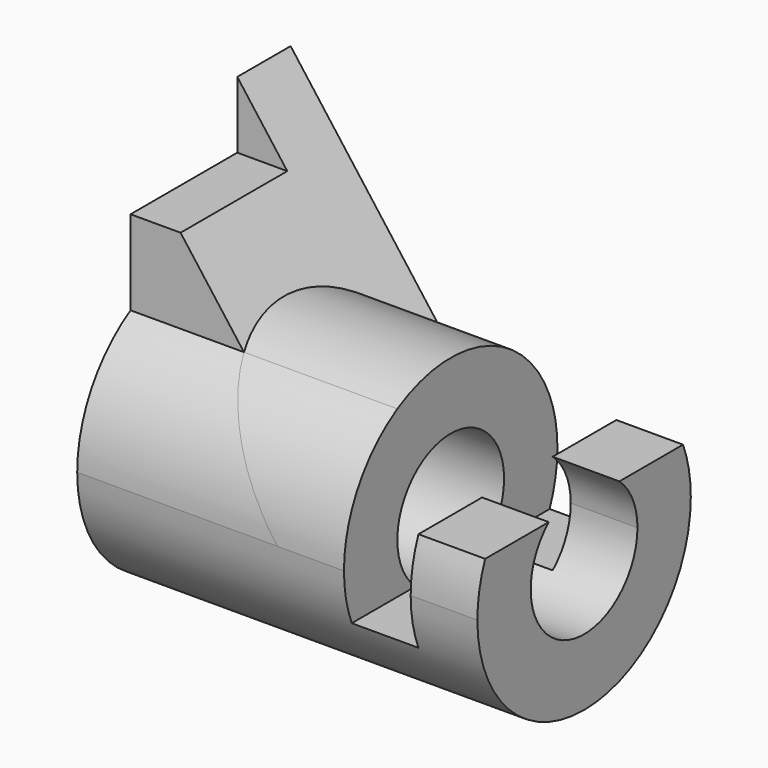
from build123d import *
from build123d import SkipClean  # not in build123d's __all__

# Parameters (mm, degrees)
F0_R      = 25.4
F1_DEPTH  = 76.2
F3_DEPTH  = 25.4
F4_W      = 12.7
F4_H      = 50.8
F5_DEPTH  = 19.05
F7_DEPTH  = 25.4
F8_R      = 12.7
F9_DEPTH  = 76.201
F11_DEPTH = 76.201
F12_W     = 25.4
F12_H     = 12.7
F13_DEPTH = 76.201


with BuildPart() as f1:
    # F0 (on Right) → F1 (new body)
    with BuildSketch(Plane.YZ):
        Circle(F0_R)
    extrude(amount=-F1_DEPTH)

    # F2 (on face) → F3 (cut)
    with BuildSketch(Plane.YZ):
        with BuildLine():
            ThreePointArc((23.5464301965, 9.525), (0, 25.4), (-23.5464301965, 9.525))
            Line((-23.5464301965, 9.525), (23.5464301965, 9.525))
        make_face()
    extrude(amount=-F3_DEPTH, mode=Mode.SUBTRACT)

    # F4 (on face) → F5 (cut)
    with BuildSketch(Plane.XY.offset(9.525)):
        with Locations((-19.05, 0)):
            Rectangle(F4_W, F4_H)
    extrude(amount=-F5_DEPTH, mode=Mode.SUBTRACT)

    # F6 (on Front) → F7 (join, symmetric)
    with BuildSketch(Plane.XZ):
        Polygon((-76.2, 0), (-38.1, 0), (-54.76875, 22.225), (-76.2, 22.225), align=None)
        Polygon((-76.2, 22.225), (-54.76875, 22.225), (-76.2, 50.8), align=None)
    extrude(amount=F7_DEPTH, both=True)

    # F8 (on Right) → F9 (cut, through all)
    with BuildSketch(Plane.YZ):
        Circle(F8_R)
    extrude(amount=-F9_DEPTH, mode=Mode.SUBTRACT)

    # F10 (on face) → F11 (cut, through all)
    with BuildSketch(Plane.YZ):
        with BuildLine():
            ThreePointArc((-25.4, 0), (-21.9970452561, 12.7), (-12.7, 21.9970452561))
            Line((-12.7, 21.9970452561), (-12.7, 50.8))
            Line((-12.7, 50.8), (-25.4, 50.8))
            Line((-25.4, 50.8), (-25.4, 0))
        make_face()
    with SkipClean():  # cleaning this boolean's faces spoils the solid; the shape is the same uncleaned
        extrude(amount=-F11_DEPTH, mode=Mode.SUBTRACT)

    # F12 (on face) → F13 (cut, through all)
    with BuildSketch(Plane.YZ):
        with Locations((0, 44.45)):
            Rectangle(F12_W, F12_H)
    with SkipClean():  # cleaning this boolean's faces spoils the solid; the shape is the same uncleaned
        extrude(amount=-F13_DEPTH, mode=Mode.SUBTRACT)


solid = f1.part
